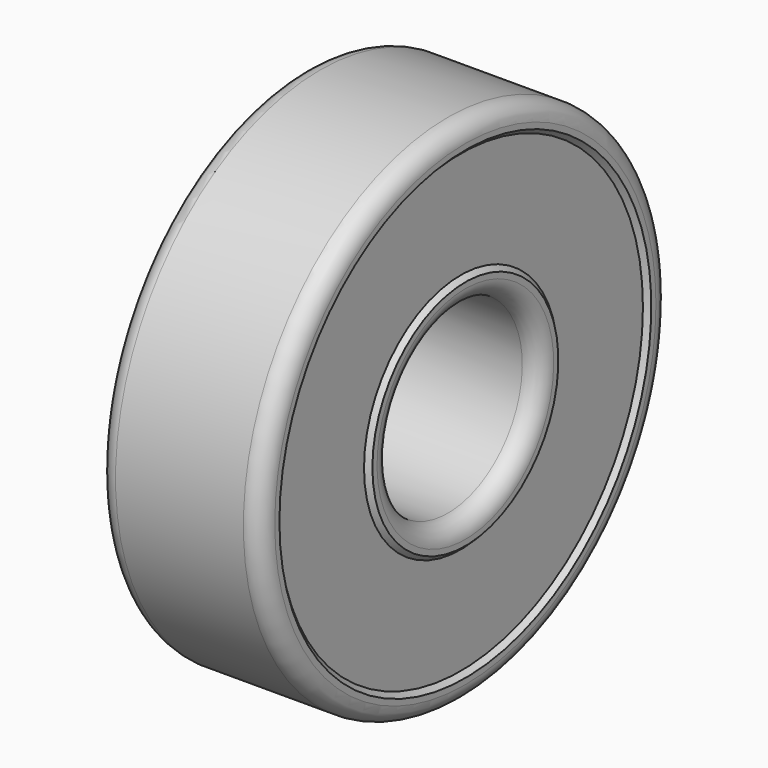
from build123d import *

# Parameters (mm, degrees)
F0_W    = 7
F0_H    = 7
F2_R    = 0.75
F3_W    = 0.2
F3_H    = 5
F5_SIZE = 0.19999


# Not quite as in the source:
# - a fillet or chamfer is up to 0.001 mm smaller than in the source, because OpenCascade refuses the exact size


with BuildPart() as f1:
    # F0 (on Front) → F1 (revolve)
    with BuildSketch(Plane.XZ):
        with Locations((0, 7.5)):
            Rectangle(F0_W, F0_H)
    revolve(axis=Axis((-0.6671294104, 0, 0), (-1, 0, 0)))

    # F2
    f2_edges = [f1.edges().sort_by_distance(p)[0] for p in [
        (-3.5, 0, -11),
        (-3.5, 0, -4),
        (3.5, 0, -11),
        (3.5, 0, -4),
    ]]
    fillet(f2_edges, radius=F2_R)

    # F3 (on Top) → F4 (revolve, cut)
    with BuildSketch(Plane.XY):
        with Locations((-3.4, -7.5)):
            Rectangle(F3_W, F3_H)
        with Locations((3.4, -7.5)):
            Rectangle(F3_W, F3_H)
    revolve(axis=Axis((0.1337367576, 0, 0), (1, 0, 0)), mode=Mode.SUBTRACT)

    # F5 (size 0.2 in the source; OpenCascade refuses exactly that, so slightly less here)
    f5_edges = [f1.edges().sort_by_distance(p)[0] for p in [
        (-3.3, 10, 0),
        (-3.3, 5, 0),
        (3.3, 10, 0),
        (3.3, 5, 0),
    ]]
    chamfer(f5_edges, length=F5_SIZE)


solid = f1.part
